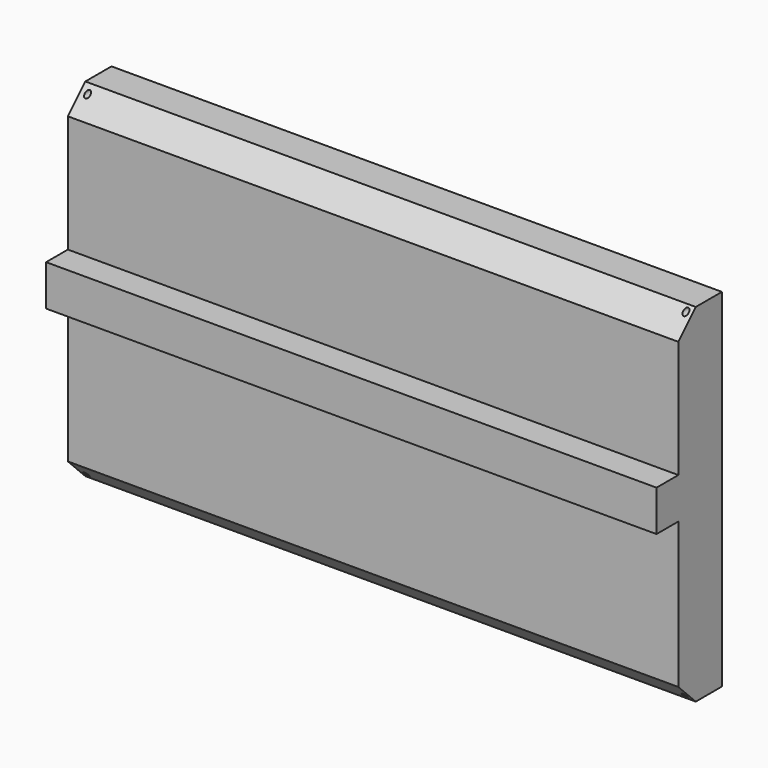
from build123d import *

# Parameters (mm, degrees)
F0_W        = 142.24
F0_H        = 80.9625
F0_R        = 0.635
F1_DEPTH    = 6.35
F2_T1_DEPTH = 168.3682991577
F3_W        = 142.24
F3_H        = 9.525
F4_DEPTH    = 6.35


# Not quite as in the source:
# - a fillet or chamfer that OpenCascade refuses, or shapes differently, is made with other operations: its cross-section is extruded or revolved along the edge and cut away or added


with BuildPart() as f1:
    # F0 (on Front) → F1 (new body, symmetric)
    with BuildSketch(Plane.XZ):
        with Locations((10.6546021998, 18.2648575297)):
            Rectangle(F0_W, F0_H)
        with Locations((-59.0889267623, -20.8356846124)):
            Circle(F0_R, mode=Mode.SUBTRACT)
        with Locations((80.2197679877, -20.9288131446)):
            Circle(F0_R, mode=Mode.SUBTRACT)
        with Locations((-58.7598197162, 57.2748109698)):
            Circle(F0_R, mode=Mode.SUBTRACT)
        with Locations((80.3315266967, 57.7001310885)):
            Circle(F0_R, mode=Mode.SUBTRACT)
    extrude(amount=F1_DEPTH, both=True)

    # F2: chamfer of 5.08 on 2 edges, made by hand

    # F2_s2 → F2_t1 (cut)
    with BuildSketch(Plane.YZ.offset(-73.5295473791)):
        Polygon((-1.27, -22.2163924703), (-6.35, -17.1363924703), (-6.35, -22.2163924703), align=None)
        Polygon((-1.27, 58.7461075297), (-6.35, 53.6661075297), (-6.35, 58.7461075297), align=None)
    extrude(amount=F2_T1_DEPTH, mode=Mode.SUBTRACT)

    # F3 (on face) → F4 (join)
    with BuildSketch(Plane.XZ.offset(6.35)):
        with Locations((10.6546021998, 21.5639811352)):
            Rectangle(F3_W, F3_H)
    extrude(amount=F4_DEPTH)


solid = f1.part
